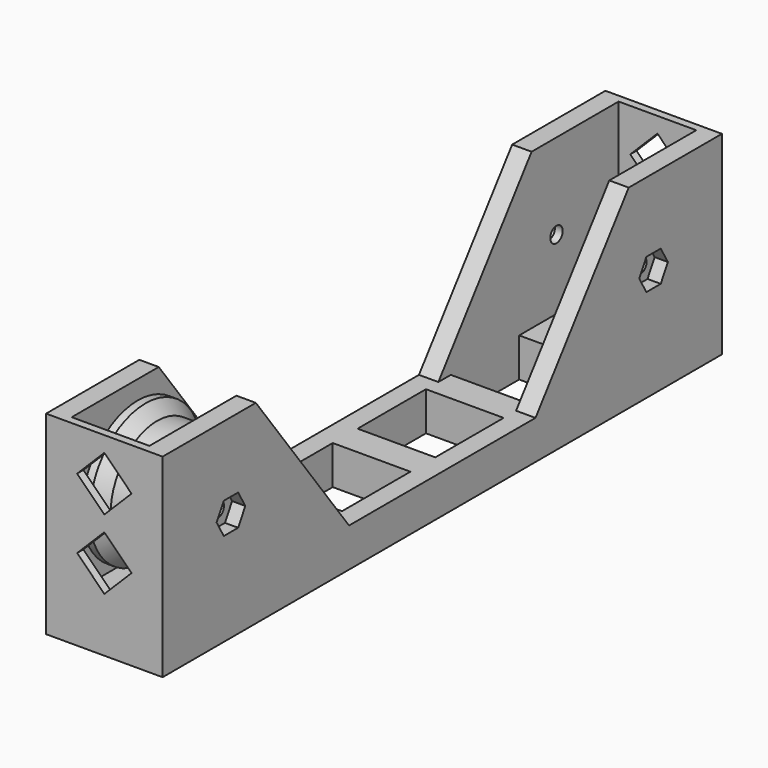
from build123d import *

# Parameters (mm, degrees)
F0_R      = 15
F1_DEPTH  = 15
F2_W      = 20
F2_H      = 30
F3_DEPTH  = 40
F2_H_2    = 58
F2_H_3    = 28
F4_DEPTH  = 40
F9_D      = 4
F9_2_D    = 4
F10_W     = 20
F10_H     = 22
F11_DEPTH = 10
F12_DEPTH = 3.4
F13_R     = 5
F14_DEPTH = 3
F16_DEPTH = 180.001


with BuildPart() as f1:
    # F0 (on Right) → F1 (new body, symmetric)
    with BuildSketch(Plane.YZ):
        Polygon((-90, 0), (0, 0), (90, 0), (90, 50), (60, 50), (30, 10), (0, 10), (-30, 10), (-60, 50), (-90, 50), align=None)
        with Locations((-68, 28)):
            Circle(F0_R, mode=Mode.SUBTRACT)
        with Locations((-68, 28)):
            Circle(F0_R)
    extrude(amount=F1_DEPTH, both=True)

    # F2 (on face) → F3 (cut, through all)
    with BuildSketch(Plane.XY.offset(50)):
        with Locations((0, -45)):
            Rectangle(F2_W, F2_H)
    extrude(amount=-F3_DEPTH, mode=Mode.SUBTRACT)

    # F2 (on face) → F4 (cut, through all)
    with BuildSketch(Plane.XY.offset(50)):
        with Locations((0, 59)):
            Rectangle(F2_W, F2_H_2)
        with Locations((0, -74)):
            Rectangle(F2_W, F2_H_3)
    extrude(amount=-F4_DEPTH, mode=Mode.SUBTRACT)

    # F9 (through all)
    with Locations(Plane.YZ.offset(15)):
        with Locations((-68, 28), (68, 28)):
            Hole(F9_D / 2)

    # F10 (on face) → F11 (cut, through all)
    with BuildSketch(Plane.XY.offset(10)):
        with Locations((0, 15)):
            Rectangle(F10_W, F10_H)
        with Locations((0, -15)):
            Rectangle(F10_W, F10_H)
        with Locations((0, -45)):
            Rectangle(F10_W, F10_H)
        with Locations((0, 45)):
            Rectangle(F10_W, F10_H)
    extrude(amount=-F11_DEPTH, mode=Mode.SUBTRACT)

    # F8 (on face) → F12 (cut, through all)
    with BuildSketch(Plane.YZ.offset(15)):
        Polygon((-70.3094010768, 24), (-65.6905989232, 24), (-63.3811978465, 28), (-65.6905989232, 32), (-70.3094010768, 32), (-72.6188021535, 28), align=None)
        Polygon((70.3094010768, 32), (65.6905989232, 32), (63.3811978465, 28), (65.6905989232, 24), (70.3094010768, 24), (72.6188021535, 28), align=None)
    extrude(amount=-F12_DEPTH, mode=Mode.SUBTRACT)

    # F13 (on face) → F14 (cut)
    with BuildSketch(Plane(origin=(-15, 0, 0), x_dir=(0, -1, 0), z_dir=(-1, 0, 0))):
        with Locations((68, 28)):
            Circle(F13_R)
        with Locations((-68, 28)):
            Circle(F13_R)
    extrude(amount=-F14_DEPTH, mode=Mode.SUBTRACT)

    # F15 (on face) → F16 (cut, through all)
    with BuildSketch(Plane(origin=(0, 90, 0), x_dir=(-1, 0, 0), z_dir=(0, 1, 0))):
        Polygon((-7, 39), (0, 32), (7, 39), (0, 46), align=None)
        Polygon((7, 21), (0, 28), (-7, 21), (0, 14), align=None)
    extrude(amount=-F16_DEPTH, mode=Mode.SUBTRACT)


with BuildPart() as f7:
    # F6 (on plane+point) → F7 (revolve)
    with BuildSketch(Plane.XZ.offset(68)):
        Polygon((4, 43), (0, 43), (-4, 43), (-7, 46), (-9, 46), (-9, 28), (0, 28), (9, 28), (9, 46), (7, 46), align=None)
    revolve(axis=Axis((-4.5, -68, 28), (1, 0, 0)))

    # F9#2 (through all)
    with Locations(Plane.YZ.offset(15)):
        with Locations((-68, 28), (68, 28)):
            Hole(F9_2_D / 2)


solid = Compound([f1.part, f7.part])
